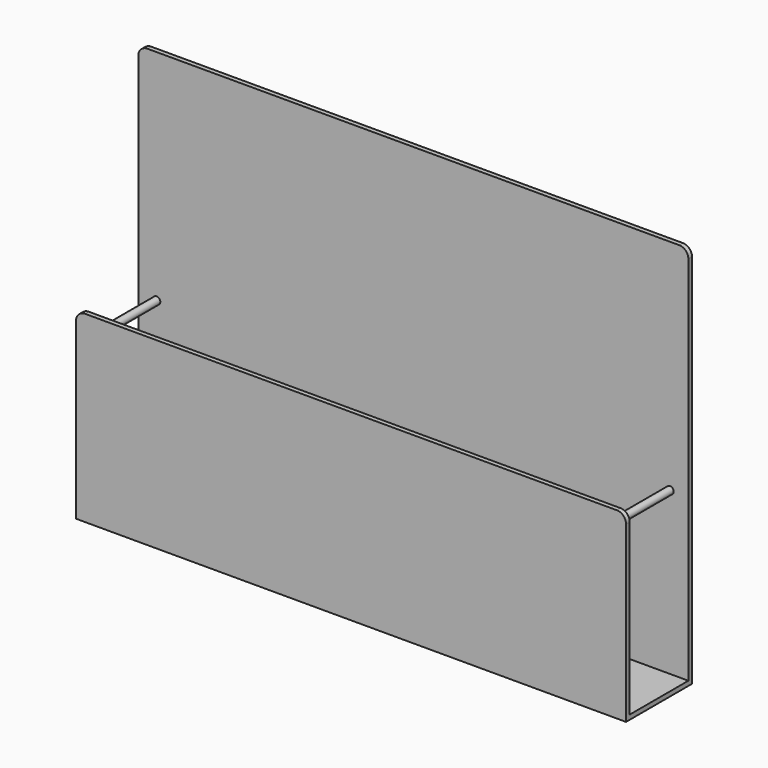
from build123d import *

# Parameters (mm, degrees)
F1_DEPTH = 5
F2_W     = 600
F2_H     = 5
F3_DEPTH = 80
F4_W     = 600
F4_H     = 5
F4_H_2   = 195
F5_DEPTH = 5
F6_R     = 10
F7_R     = 4
F8_DEPTH = 85


# Not quite as in the source:
# - a feature names something its author has since deleted; it is built from what else it names


with BuildPart() as f1:
    # F0 (on Front) → F1 (new body)
    with BuildSketch(Plane.XZ):
        with BuildLine():
            Line((26.5459360182, 400.2749490738), (-553.4540639818, 400.2749490738))
            ThreePointArc((-553.4540639818, 400.2749490738), (-560.5251317936, 397.3460168857), (-563.4540639818, 390.2749490738))
            Line((-563.4540639818, 390.2749490738), (-563.4540639818, -19.7250509262))
            Line((-563.4540639818, -19.7250509262), (36.5459360182, -19.7250509262))
            Line((36.5459360182, -19.7250509262), (36.5459360182, 390.2749490738))
            ThreePointArc((36.5459360182, 390.2749490738), (33.6170038301, 397.3460168857), (26.5459360182, 400.2749490738))
        make_face()
    extrude(amount=F1_DEPTH)

    # F2 (on face) → F3 (join)
    with BuildSketch(Plane.XZ.offset(5)):
        with Locations((-263.4540639818, -17.2250509262)):
            Rectangle(F2_W, F2_H)
    extrude(amount=F3_DEPTH)

    # F4 (on face) → F5 (join)
    with BuildSketch(Plane.XZ.offset(85)):
        with Locations((-263.4540639818, -17.2250509262)):
            Rectangle(F4_W, F4_H)
        with Locations((-263.4540639818, 82.7749490738)):
            Rectangle(F4_W, F4_H_2)
    extrude(amount=F5_DEPTH)

    # F6
    f6_edges = [f1.edges().sort_by_distance(p)[0] for p in [
        (-563.454064, -87.5, 180.274949),
        (36.545936, -87.5, 180.274949),
    ]]
    fillet(f6_edges, radius=F6_R)

    # F7 (on face) → F8 (join)
    with BuildSketch(Plane.XZ.offset(90)):
        with Locations((-543.4540639818, 161.7681980133)):
            Circle(F7_R)
        with Locations((16.5459360182, 161.7681980133)):
            Circle(F7_R)
    extrude(amount=-F8_DEPTH)


solid = f1.part
